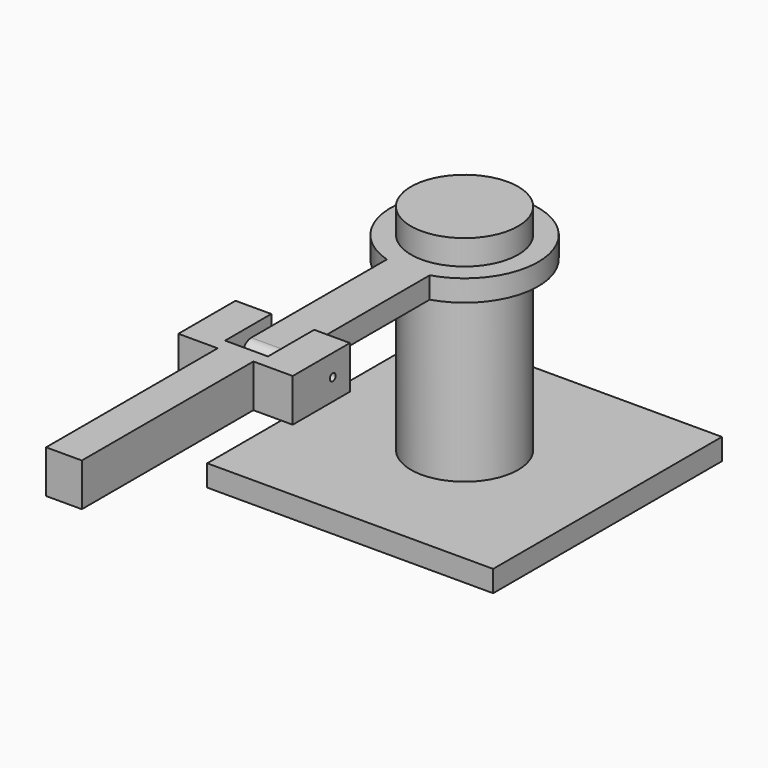
from build123d import *

# Parameters (mm, degrees)
F0_W      = 40
F0_H      = 40
F1_DEPTH  = 3
F2_R      = 7.5
F3_DEPTH  = 30
F5_R      = 7.5
F6_DEPTH  = 1.5
F8_DEPTH  = 3
F9_R      = 1.49999
F10_R     = 0.5
F11_DEPTH = 23.001
F12_R     = 0.5
F13_DEPTH = 28.001


# Not quite as in the source:
# - a fillet or chamfer is up to 0.001 mm smaller than in the source, because OpenCascade refuses the exact size


with BuildPart() as f1:
    # F0 (on Top) → F1 (new body)
    with BuildSketch(Plane.XY):
        Rectangle(F0_W, F0_H)
    extrude(amount=-F1_DEPTH)


with BuildPart() as f3:
    # F2 (on face) → F3 (new body)
    with BuildSketch(Plane.XY):
        Circle(F2_R)
    extrude(amount=F3_DEPTH)


with BuildPart() as f6:
    # F5 (on offset) → F6 (new body, symmetric)
    with BuildSketch(Plane.XY.offset(25)):
        with BuildLine():
            Line((3, -35.0465811789), (3, -9.846652891))
            ThreePointArc((3, -9.846652891), (0, 10.2935209309), (-3, -9.846652891))
            Line((-3, -9.846652891), (-3, -35.0465811789))
            Line((-3, -35.0465811789), (3, -35.0465811789))
        make_face()
        Circle(F5_R, mode=Mode.SUBTRACT)
    extrude(amount=-F6_DEPTH, both=True)

    # F9 (radius 1.5 in the source; OpenCascade refuses exactly that, so slightly less here)
    f9_edges = [f6.edges().sort_by_distance(p)[0] for p in [
        (0, -35.046581, 23.5),
        (0, -35.046581, 26.5),
    ]]
    fillet(f9_edges, radius=F9_R)

    # F10 (on face) → F11 (cut, through all)
    with BuildSketch(Plane(origin=(-3, 0, 0), x_dir=(0, -1, 0), z_dir=(-1, 0, 0))):
        with Locations((33.5465811789, 25)):
            Circle(F10_R)
    extrude(amount=-F11_DEPTH, mode=Mode.SUBTRACT)


with BuildPart() as f8:
    # F7 (on offset) → F8 (new body, symmetric)
    with BuildSketch(Plane.XY.offset(25)):
        Polygon((-3, -35.0465811789), (-3, -30.0465811789), (-8, -30.0465811789), (-8, -40.0465811789), (-2.5, -40.0465811789), (-2.5, -70.0465811789), (2.5, -70.0465811789), (2.5, -40.0465811789), (8, -40.0465811789), (8, -30.0465811789), (3, -30.0465811789), (3, -35.0465811789), (3, -38.1220765412), (-3, -38.1220765412), align=None)
    extrude(amount=F8_DEPTH, both=True)

    # F12 (on face) → F13 (cut, through all)
    with BuildSketch(Plane(origin=(-8, 0, 0), x_dir=(0, -1, 0), z_dir=(-1, 0, 0))):
        with Locations((33.0465811789, 25)):
            Circle(F12_R)
    extrude(amount=-F13_DEPTH, mode=Mode.SUBTRACT)


solid = Compound([f1.part, f3.part, f6.part, f8.part])
